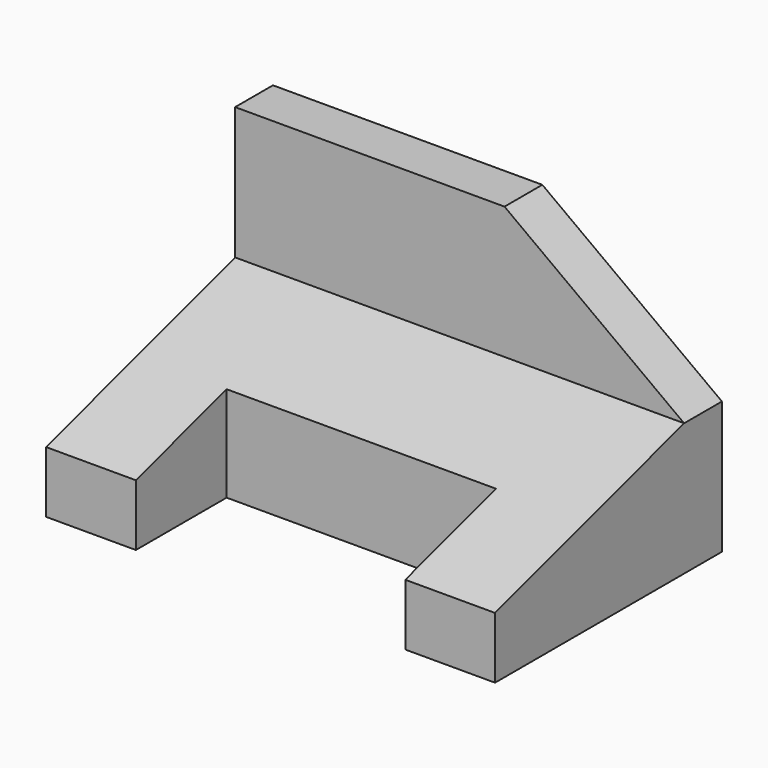
from build123d import *

# Parameters (mm, degrees)
F1_DEPTH = 95
F3_DEPTH = 10.001
F4_W     = 57
F4_H     = 24
F6_DEPTH = 180
F7_W     = 57
F7_H     = 24
F8_DEPTH = 56.001
F9_DEPTH = 179


# Not quite as in the source:
# - an extrude ends at something that could not be found from the text; its depth is read off the source's solid
# - a feature of the source that left no trace in its solid (it failed there, or was rolled back) is left out
# - a feature names something its author has since deleted; it is built from what else it names


with BuildPart() as f1:
    # F0 (on Right) → F1 (new body)
    with BuildSketch(Plane.YZ):
        Polygon((0, 56), (-10, 56), (-10, 28), (-60, 13), (-60, 0), (0, 0), align=None)
    extrude(amount=F1_DEPTH)

    # F2 (on face) → F3 (cut, through all)
    with BuildSketch(Plane.XZ.offset(10)):
        Polygon((95, 56), (57, 56), (95, 28), align=None)
    extrude(amount=-F3_DEPTH, mode=Mode.SUBTRACT)

    # F4 (on face) → F6 (cut, through all)
    with BuildSketch(Plane(origin=(0, 0, 0), x_dir=(1, 0, 0), z_dir=(0, 0, -1))):
        with Locations((47.5, 48)):
            Rectangle(F4_W, F4_H)
    extrude(amount=F6_DEPTH, mode=Mode.SUBTRACT)

    # F7 (on face) → F8 (cut, through all)
    with BuildSketch(Plane(origin=(0, 0, 0), x_dir=(1, 0, 0), z_dir=(0, 0, -1))):
        with Locations((47.5, 48)):
            Rectangle(F7_W, F7_H)
    extrude(amount=-F8_DEPTH, mode=Mode.SUBTRACT)

    # F4 (on face) → F9 (cut, through all)
    with BuildSketch(Plane(origin=(0, 0, 0), x_dir=(1, 0, 0), z_dir=(0, 0, -1))):
        with Locations((47.5, 48)):
            Rectangle(F4_W, F4_H)
    extrude(amount=F9_DEPTH, mode=Mode.SUBTRACT)


solid = f1.part
